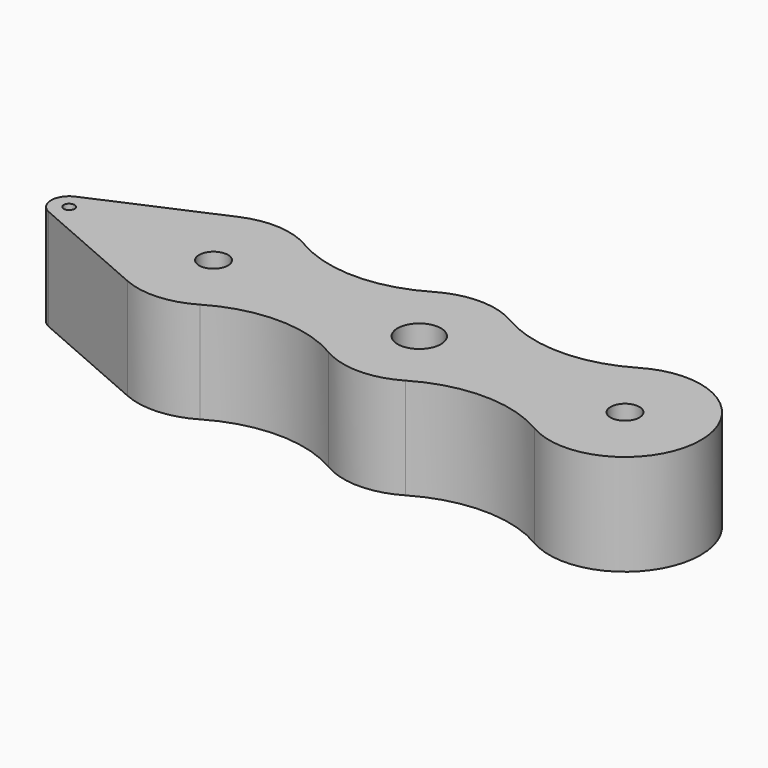
from build123d import *

# Parameters (mm, degrees)
F0_R     = 1.5
F0_R_2   = 4
F0_R_3   = 6
F1_DEPTH = 28


# Not quite as in the source:
# - ends of sketch curves that miss each other by under 0.0002 mm in the source are joined


with BuildPart() as f1:
    # F0 (on Top) → F1 (new body)
    with BuildSketch(Plane.XY):
        with BuildLine():
            ThreePointArc((-46.3352200183, -18.0903971195), (-28.5000011764, -13.2245283483), (-10.6647820085, -18.0903959247))
            ThreePointArc((-10.6647820085, -18.0903959247), (21, 0), (-10.6647820085, 18.0903959247))
            ThreePointArc((-10.6647820085, 18.0903959247), (-28.5000011764, 13.2245283483), (-46.3352200183, 18.0903971195))
            ThreePointArc((-46.3352200183, 18.0903971195), (-57.0000007926, 21), (-67.6647813473, 18.0903963145))
            ThreePointArc((-67.6647813473, 18.0903963145), (-85.5000011764, 13.2245283483), (-103.3352200183, 18.0903971195))
            ThreePointArc((-103.3352200183, 18.0903971195), (-112.7285298393, 20.9614733173), (-122.4, 19.2468179188))
            Line((-122.4, 19.2468179188), (-156, 4.582575695))
            ThreePointArc((-156, 4.582575695), (-159, 0), (-156, -4.582575695))
            Line((-156, -4.582575695), (-122.4, -19.2468179188))
            ThreePointArc((-122.4, -19.2468179188), (-112.7285306305, -20.9614733653), (-103.3352200183, -18.0903971195))
            ThreePointArc((-103.3352200183, -18.0903971195), (-85.5000011764, -13.2245283483), (-67.6647820085, -18.0903959247))
            ThreePointArc((-67.6647820085, -18.0903959247), (-57.0000011764, -21), (-46.3352200183, -18.0903971195))
        make_face()
        with Locations((-154, 0)):
            Circle(F0_R, mode=Mode.SUBTRACT)
        with Locations((-114, 0)):
            Circle(F0_R_2, mode=Mode.SUBTRACT)
        with Locations((-57, 0)):
            Circle(F0_R_3, mode=Mode.SUBTRACT)
        Circle(F0_R_2, mode=Mode.SUBTRACT)
    extrude(amount=F1_DEPTH)


solid = f1.part
